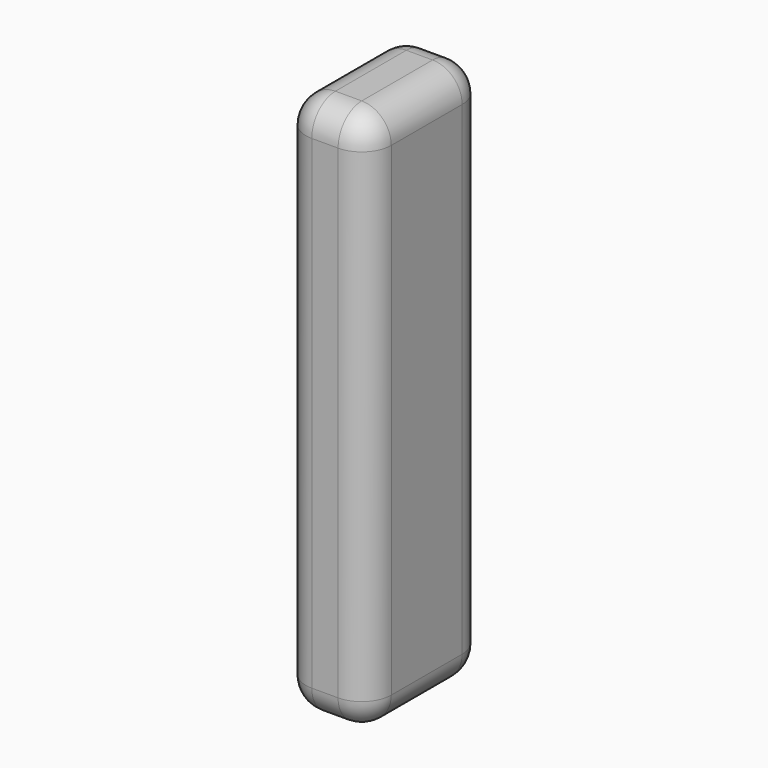
from build123d import *

# Parameters (mm, degrees)
F0_W         = 14.6878659725
F0_H         = 93.4034362435
F1_DEPTH     = 25.4
F2_R         = 5.08
F3_R         = 5.08
F4_T1_DEPTH  = 4.5278659725
F4_T3_DEPTH  = 15.24
F4_S7_W      = 5.08
F4_S7_H      = 5.08
F4_T8_DEPTH  = 5.08
F4_S13_W     = 5.08
F4_S13_H     = 5.08
F4_T14_DEPTH = 5.08
F4_S19_W     = 5.08
F4_S19_H     = 5.08
F4_T20_DEPTH = 5.08
F4_S25_W     = 5.08
F4_S25_H     = 5.08
F4_T26_DEPTH = 5.08
F4_T30_ANGLE = 90
F4_T32_ANGLE = 90
F4_T34_ANGLE = 90
F4_T36_ANGLE = 90


# Not quite as in the source:
# - a fillet or chamfer that OpenCascade refuses, or shapes differently, is made with other operations: its cross-section is extruded or revolved along the edge and cut away or added


with BuildPart() as f1:
    # F0 (on Front) → F1 (new body)
    with BuildSketch(Plane.XZ):
        with Locations((7.3439329863, -46.7017181218)):
            Rectangle(F0_W, F0_H)
    extrude(amount=F1_DEPTH)

    # F2
    f2_edges = [f1.edges().sort_by_distance(p)[0] for p in [
        (14.687866, -25.4, -46.701718),
        (7.343933, -25.4, 0),
        (0, -25.4, -46.701718),
        (7.343933, -25.4, -93.403436),
    ]]
    fillet(f2_edges, radius=F2_R)

    # F3
    f3_edges = [f1.edges().sort_by_distance(p)[0] for p in [
        (14.687866, 0, -46.701718),
        (0, 0, -46.701718),
    ]]
    fillet(f3_edges, radius=F3_R)

    # F4: fillet of radius 5.08 on 2 edges, made by hand

    # F4_s2 → F4_t1 (cut)
    with BuildSketch(Plane.YZ.offset(5.08)):
        with BuildLine():
            ThreePointArc((0, -88.3234362435), (-1.4878975516, -91.915538692), (-5.08, -93.4034362435))
            Line((-5.08, -93.4034362435), (0, -93.4034362435))
            Line((0, -93.4034362435), (0, -88.3234362435))
        make_face()
        with BuildLine():
            ThreePointArc((-5.08, 0), (-1.4878975516, -1.4878975516), (0, -5.08))
            Line((0, -5.08), (0, 0))
            Line((0, 0), (-5.08, 0))
        make_face()
    extrude(amount=F4_T1_DEPTH, mode=Mode.SUBTRACT)

    # F4_s4 → F4_t3 (cut)
    with BuildSketch(Plane.XZ.offset(5.08)):
        with BuildLine():
            ThreePointArc((5.08, 0), (1.4878975516, -1.4878975516), (0, -5.08))
            Line((0, -5.08), (0, 0))
            Line((0, 0), (5.08, 0))
        make_face()
        with BuildLine():
            ThreePointArc((9.6078659725, 0), (13.1999684209, -1.4878975516), (14.6878659725, -5.08))
            Line((14.6878659725, -5.08), (14.6878659725, 0))
            Line((14.6878659725, 0), (9.6078659725, 0))
        make_face()
        with BuildLine():
            ThreePointArc((14.6878659725, -88.3234362435), (13.1999684209, -91.915538692), (9.6078659725, -93.4034362435))
            Line((9.6078659725, -93.4034362435), (14.6878659725, -93.4034362435))
            Line((14.6878659725, -93.4034362435), (14.6878659725, -88.3234362435))
        make_face()
        with BuildLine():
            ThreePointArc((0, -88.3234362435), (1.4878975516, -91.915538692), (5.08, -93.4034362435))
            Line((5.08, -93.4034362435), (0, -93.4034362435))
            Line((0, -93.4034362435), (0, -88.3234362435))
        make_face()
    extrude(amount=F4_T3_DEPTH, mode=Mode.SUBTRACT)


with BuildPart() as f4_tool6:
    # F4_s7 → F4_t8 (new body)
    with BuildSketch(Plane.XY.offset(-5.08)):
        with Locations((2.54, -22.86)):
            Rectangle(F4_S7_W, F4_S7_H)
    extrude(amount=F4_T8_DEPTH)

    # F4_s9 → F4_t10 (revolve, cut)
    with BuildSketch(Plane(origin=(5.08, -20.32, -5.08), x_dir=(0.7071067812, 0.7071067812, 0), z_dir=(0.7071067812, -0.7071067812, 0))):
        with BuildLine():
            ThreePointArc((0, -5.08), (5.08, 0), (0, 5.08))
            Line((0, 5.08), (0, -5.08))
        make_face()
    revolve(axis=Axis((5.08, -20.32, -5.08), (0, 0, 1)), mode=Mode.SUBTRACT)


with BuildPart() as f1_1:
    add(f1.part)

    # F4_t5: cut F4_tool6
    add(f4_tool6.part, mode=Mode.SUBTRACT)


with BuildPart() as f4_tool12:
    # F4_s13 → F4_t14 (new body)
    with BuildSketch(Plane.XY.offset(-5.08)):
        with Locations((12.1478659725, -22.86)):
            Rectangle(F4_S13_W, F4_S13_H)
    extrude(amount=F4_T14_DEPTH)

    # F4_s15 → F4_t16 (revolve, cut)
    with BuildSketch(Plane(origin=(9.6078659725, -20.32, -5.08), x_dir=(-0.7071067812, 0.7071067812, 0), z_dir=(0.7071067812, 0.7071067812, 0))):
        with BuildLine():
            ThreePointArc((0, -5.08), (5.08, 0), (0, 5.08))
            Line((0, 5.08), (0, -5.08))
        make_face()
    revolve(axis=Axis((9.6078659725, -20.32, -5.08), (0, 0, 1)), mode=Mode.SUBTRACT)


with BuildPart() as f1_2:
    add(f1_1.part)

    # F4_t11: cut F4_tool12
    add(f4_tool12.part, mode=Mode.SUBTRACT)


with BuildPart() as f4_tool18:
    # F4_s19 → F4_t20 (new body)
    with BuildSketch(Plane.YZ.offset(9.6078659725)):
        with Locations((-22.86, -90.8634362435)):
            Rectangle(F4_S19_W, F4_S19_H)
    extrude(amount=F4_T20_DEPTH)

    # F4_s21 → F4_t22 (revolve, cut)
    with BuildSketch(Plane(origin=(9.6078659725, -20.32, -88.3234362435), x_dir=(0, 0.7071067812, 0.7071067812), z_dir=(0, 0.7071067812, -0.7071067812))):
        with BuildLine():
            ThreePointArc((0, -5.08), (5.08, 0), (0, 5.08))
            Line((0, 5.08), (0, -5.08))
        make_face()
    revolve(axis=Axis((9.6078659725, -20.32, -88.3234362435), (1, 0, 0)), mode=Mode.SUBTRACT)


with BuildPart() as f1_3:
    add(f1_2.part)

    # F4_t17: cut F4_tool18
    add(f4_tool18.part, mode=Mode.SUBTRACT)


with BuildPart() as f4_tool24:
    # F4_s25 → F4_t26 (new body)
    with BuildSketch(Plane.YZ.offset(5.08)):
        with Locations((-22.86, -90.8634362435)):
            Rectangle(F4_S25_W, F4_S25_H)
    extrude(amount=-F4_T26_DEPTH)

    # F4_s27 → F4_t28 (revolve, cut)
    with BuildSketch(Plane(origin=(5.08, -20.32, -88.3234362435), x_dir=(0, 0.7071067812, 0.7071067812), z_dir=(0, -0.7071067812, 0.7071067812))):
        with BuildLine():
            ThreePointArc((0, -5.08), (5.08, 0), (0, 5.08))
            Line((0, 5.08), (0, -5.08))
        make_face()
    revolve(axis=Axis((5.08, -20.32, -88.3234362435), (-1, 0, 0)), mode=Mode.SUBTRACT)


with BuildPart() as f1_4:
    add(f1_3.part)

    # F4_t23: cut F4_tool24
    add(f4_tool24.part, mode=Mode.SUBTRACT)

    # F4_s29 → F4_t30 (revolve, cut)
    with BuildSketch(Plane.XZ.offset(5.08)):
        with BuildLine():
            ThreePointArc((9.6078659725, 0), (13.1999684209, -1.4878975516), (14.6878659725, -5.08))
            Line((14.6878659725, -5.08), (14.6878659725, 0))
            Line((14.6878659725, 0), (9.6078659725, 0))
        make_face()
    revolve(axis=Axis((9.6078659725, -5.08, 0), (0, 0, 1)), revolution_arc=F4_T30_ANGLE, mode=Mode.SUBTRACT)

    # F4_s31 → F4_t32 (revolve, cut)
    with BuildSketch(Plane.YZ.offset(5.08)):
        with BuildLine():
            ThreePointArc((-5.08, 0), (-1.4878975516, -1.4878975516), (0, -5.08))
            Line((0, -5.08), (0, 0))
            Line((0, 0), (-5.08, 0))
        make_face()
    revolve(axis=Axis((5.08, -5.08, 0), (0, 0, 1)), revolution_arc=F4_T32_ANGLE, mode=Mode.SUBTRACT)

    # F4_s33 → F4_t34 (revolve, cut)
    with BuildSketch(Plane.YZ.offset(5.08)):
        with BuildLine():
            ThreePointArc((0, -88.3234362435), (-1.4878975516, -91.915538692), (-5.08, -93.4034362435))
            Line((-5.08, -93.4034362435), (0, -93.4034362435))
            Line((0, -93.4034362435), (0, -88.3234362435))
        make_face()
    revolve(axis=Axis((5.08, -5.08, -93.4034362435), (0, 0, 1)), revolution_arc=F4_T34_ANGLE, mode=Mode.SUBTRACT)

    # F4_s35 → F4_t36 (revolve, cut)
    with BuildSketch(Plane.XZ.offset(5.08)):
        with BuildLine():
            ThreePointArc((14.6878659725, -88.3234362435), (13.1999684209, -91.915538692), (9.6078659725, -93.4034362435))
            Line((9.6078659725, -93.4034362435), (14.6878659725, -93.4034362435))
            Line((14.6878659725, -93.4034362435), (14.6878659725, -88.3234362435))
        make_face()
    revolve(axis=Axis((9.6078659725, -5.08, -93.4034362435), (0, 0, 1)), revolution_arc=F4_T36_ANGLE, mode=Mode.SUBTRACT)


solid = f1_4.part
